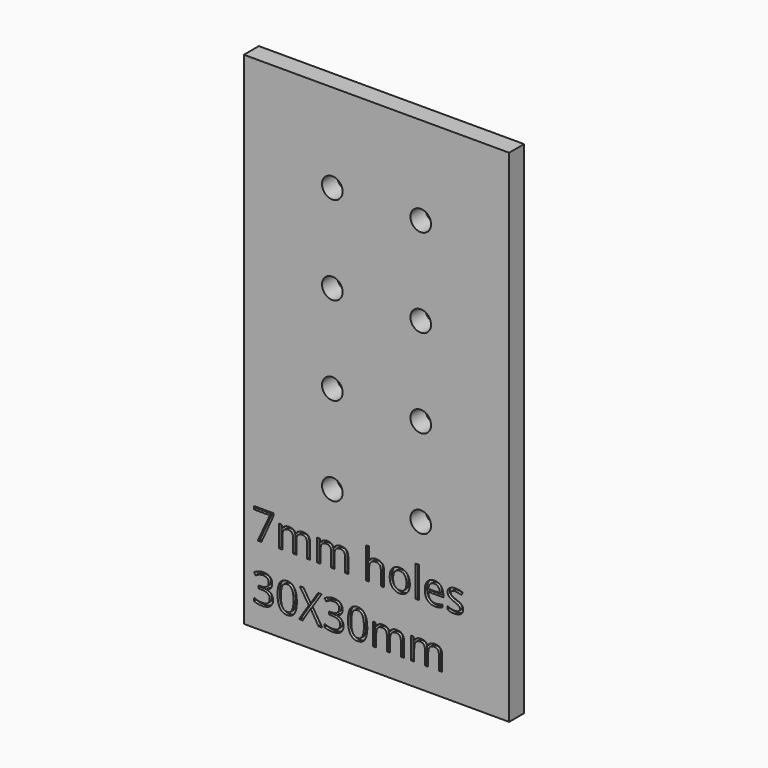
from build123d import *

# Parameters (mm, degrees)
F0_W         = 90
F0_H         = 170
F0_R         = 3.5
F1_DEPTH     = 6.35
F0_R_2       = 1.5
F3_TEXT_SIZE = 13.8888888889
F4_DEPTH     = 1


# Not quite as in the source:
# - Text() gives the source's letters only with a copy of the font that has no kerning and outlines rounded to 1/6400 em; it was checked with that copy


with BuildPart() as f1:
    # F0 (on Front) → F1 (new body)
    with BuildSketch(Plane.XZ):
        Rectangle(F0_W, F0_H)
        with Locations((-15, -35)):
            Circle(F0_R, mode=Mode.SUBTRACT)
        with Locations((-15, -5)):
            Circle(F0_R, mode=Mode.SUBTRACT)
        with Locations((15, -35)):
            Circle(F0_R, mode=Mode.SUBTRACT)
        with Locations((15, -5)):
            Circle(F0_R, mode=Mode.SUBTRACT)
        with Locations((-15, 25)):
            Circle(F0_R, mode=Mode.SUBTRACT)
        with Locations((15, 25)):
            Circle(F0_R, mode=Mode.SUBTRACT)
        with Locations((-15, 55)):
            Circle(F0_R, mode=Mode.SUBTRACT)
        with Locations((15, 55)):
            Circle(F0_R, mode=Mode.SUBTRACT)
    extrude(amount=F1_DEPTH)

    # F3 (on face) → F4 (cut)
    with BuildSketch(Plane.XZ.offset(6.35)):
        with Locations((-42.2153026565, -58.5770174503)):
            Text('7mm holes', F3_TEXT_SIZE, font='Open Sans', text_align=(TextAlign.LEFT, TextAlign.BOTTOM))
        with Locations((-42.2153026565, -77.4659063392)):
            Text('30X30mm', F3_TEXT_SIZE, font='Open Sans', text_align=(TextAlign.LEFT, TextAlign.BOTTOM))
    extrude(amount=-F4_DEPTH, mode=Mode.SUBTRACT)


with BuildPart() as f1b:
    # F0 (on Front) → F1, piece 2 (new body)
    with BuildSketch(Plane.XZ):
        with Locations((-415, 250)):
            Circle(F0_R_2)
    extrude(amount=F1_DEPTH)


solid = f1.part
